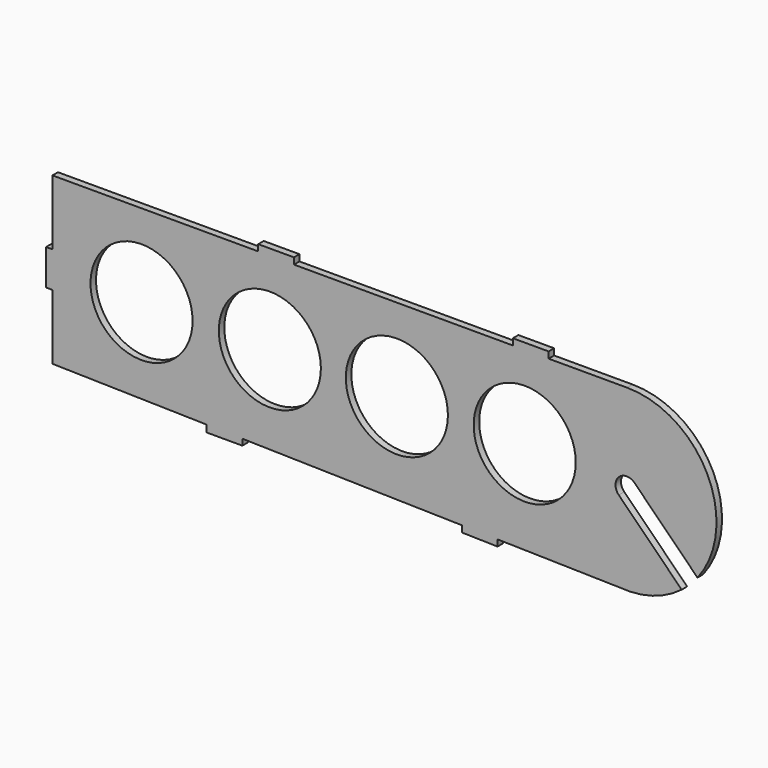
from build123d import *

# Parameters (mm, degrees)
F0_R     = 25.4
F1_DEPTH = 3.429


# Not quite as in the source:
# - ends of sketch curves that miss each other by under 0.0002 mm in the source are joined


with BuildPart() as f1:
    # F0 (on Front) → F1 (new body)
    with BuildSketch(Plane.XZ):
        with BuildLine():
            ThreePointArc((41.7896266471, 178.027378047), (41.789613947, 185.885114853), (49.647350753, 185.8851021529))
            Line((49.647350753, 185.8851021529), (80.9744634, 154.557984))
            ThreePointArc((80.9744634, 154.557984), (85.932800118, 201.4235329487), (45.972476, 226.4062528))
            Line((45.972476, 226.4062528), (6.888226, 226.4062528))
            Line((6.888226, 226.4062528), (6.888226, 229.5812528))
            Line((6.888226, 229.5812528), (-10.891774, 229.5812528))
            Line((-10.891774, 229.5812528), (-10.891774, 226.4062528))
            Line((-10.891774, 226.4062528), (-119.857774, 226.4062528))
            Line((-119.857774, 226.4062528), (-119.857774, 229.5812528))
            Line((-119.857774, 229.5812528), (-137.637774, 229.5812528))
            Line((-137.637774, 229.5812528), (-137.637774, 226.4062528))
            Line((-137.637774, 226.4062528), (-240.031524, 226.4062528))
            Line((-240.031524, 226.4062528), (-240.031524, 194.0212528))
            Line((-240.031524, 194.0212528), (-243.206524, 194.0212528))
            Line((-243.206524, 194.0212528), (-243.206524, 176.2412528))
            Line((-243.206524, 176.2412528), (-240.031524, 176.2412528))
            Line((-240.031524, 176.2412528), (-240.031524, 143.8562528))
            Line((-240.031524, 143.8562528), (-163.323524, 142.1719534))
            Line((-163.323524, 142.1719534), (-163.323524, 138.7199156))
            Line((-163.323524, 138.7199156), (-145.543524, 138.7199156))
            Line((-145.543524, 138.7199156), (-145.543524, 141.7815554))
            Line((-145.543524, 141.7815554), (-36.2456222, 139.3816618))
            Line((-36.2456222, 139.3816618), (-36.3153198, 136.2074238))
            Line((-36.3153198, 136.2074238), (-18.5353198, 135.8170258))
            Line((-18.5353198, 135.8170258), (-18.4656222, 138.9912638))
            Line((-18.4656222, 138.9912638), (47.67707, 137.5389426))
            ThreePointArc((47.67707, 137.5389426), (61.0963656021, 140.1582808001), (73.0847311317, 146.7322819609))
            Line((73.0847311317, 146.7322819609), (41.7896266471, 178.027378047))
        make_face()
        with Locations((-195.7019962, 185.2907394)):
            Circle(F0_R, mode=Mode.SUBTRACT)
        with Locations((-131.8551084, 185.2907394)):
            Circle(F0_R, mode=Mode.SUBTRACT)
        with Locations((-68.6405282, 185.2907394)):
            Circle(F0_R, mode=Mode.SUBTRACT)
        with Locations((-5.0234596, 185.2907394)):
            Circle(F0_R, mode=Mode.SUBTRACT)
    extrude(amount=F1_DEPTH)


solid = f1.part
